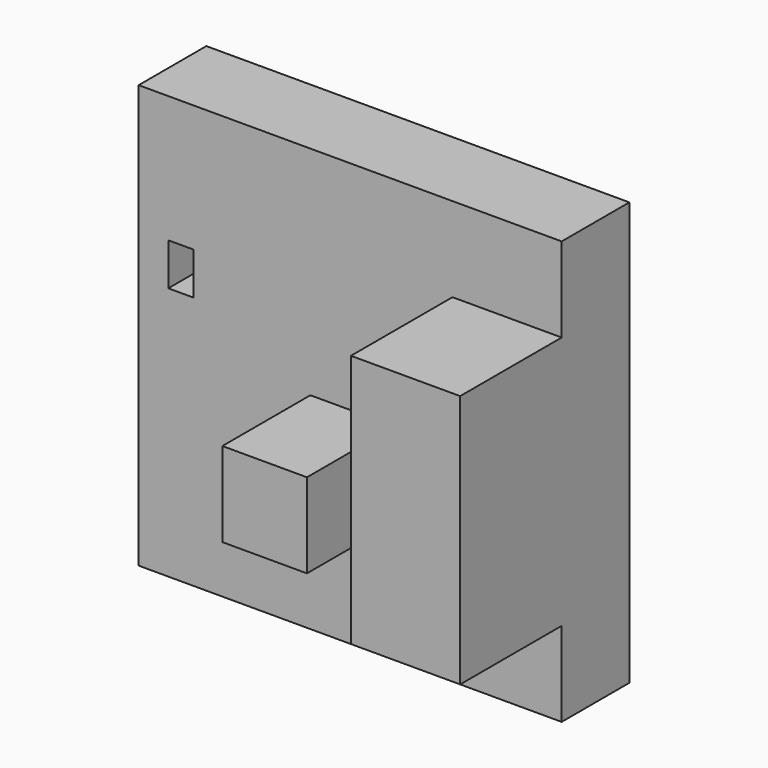
from build123d import *

# Parameters (mm, degrees)
F0_W      = 12.9061160609
F0_H      = 30
F1_DEPTH  = 25
F2_DEPTH  = 10
F3_W      = 6.5
F3_H      = 10
F4_DEPTH  = 10
F5_W      = 6.5
F5_H      = 10
F6_DEPTH  = 10
F7_W      = 15
F7_H      = 30
F8_DEPTH  = 22.9061160609
F9_W      = 10
F9_H      = 10
F10_DEPTH = 6.5
F11_W     = 3
F11_H     = 5
F12_DEPTH = 10


with BuildPart() as f1:
    # F0 (on Front) → F1 (new body)
    with BuildSketch(Plane.XZ):
        with Locations((18.5469419695, 0)):
            Rectangle(F0_W, F0_H)
    extrude(amount=F1_DEPTH)



with BuildPart() as f1b:
    # F0 (on Front) → F1, piece 2 (new body)
    with BuildSketch(Plane.XZ):
        with Locations((-18.5469419695, 0)):
            Rectangle(F0_W, F0_H)
    extrude(amount=F1_DEPTH)


with BuildPart() as f1_1:
    add(f1.part)

    add(f1b.part)  # F2 merges F1b
    # F0 (on Front) → F2 (join)
    with BuildSketch(Plane.XZ):
        Polygon((25, 15), (25, 25), (-25, 25), (-25, 15), (-12.0938839391, 15), (-12.0938839391, -15), (-25, -15), (-25, -25), (25, -25), (25, -15), (12.0938839391, -15), (12.0938839391, 15), align=None)
    extrude(amount=F2_DEPTH)

    # F3 (on face) → F4 (join)
    with BuildSketch(Plane.YZ.offset(-12.0938839391)):
        with Locations((-21.75, 0)):
            Rectangle(F3_W, F3_H)
    extrude(amount=F4_DEPTH)

    # F5 (on face) → F6 (join)
    with BuildSketch(Plane(origin=(12.0938839391, 0, 0), x_dir=(0, -1, 0), z_dir=(-1, 0, 0))):
        with Locations((21.75, 0)):
            Rectangle(F5_W, F5_H)
    extrude(amount=F6_DEPTH)

    # F7 (on face) → F8 (cut, through all)
    with BuildSketch(Plane(origin=(-25, 0, 0), x_dir=(0, -1, 0), z_dir=(-1, 0, 0))):
        with Locations((17.5, 0)):
            Rectangle(F7_W, F7_H)
    extrude(amount=-F8_DEPTH, mode=Mode.SUBTRACT)

    # F9 (on face) → F10 (join)
    with BuildSketch(Plane.XZ.offset(25)):
        with Locations((7.0938839391, 0)):
            Rectangle(F9_W, F9_H)
    extrude(amount=F10_DEPTH)

    # F11 (on face) → F12 (cut)
    with BuildSketch(Plane.XZ.offset(10)):
        with Locations((-20, 7.5)):
            Rectangle(F11_W, F11_H)
    extrude(amount=-F12_DEPTH, mode=Mode.SUBTRACT)


solid = f1_1.part
